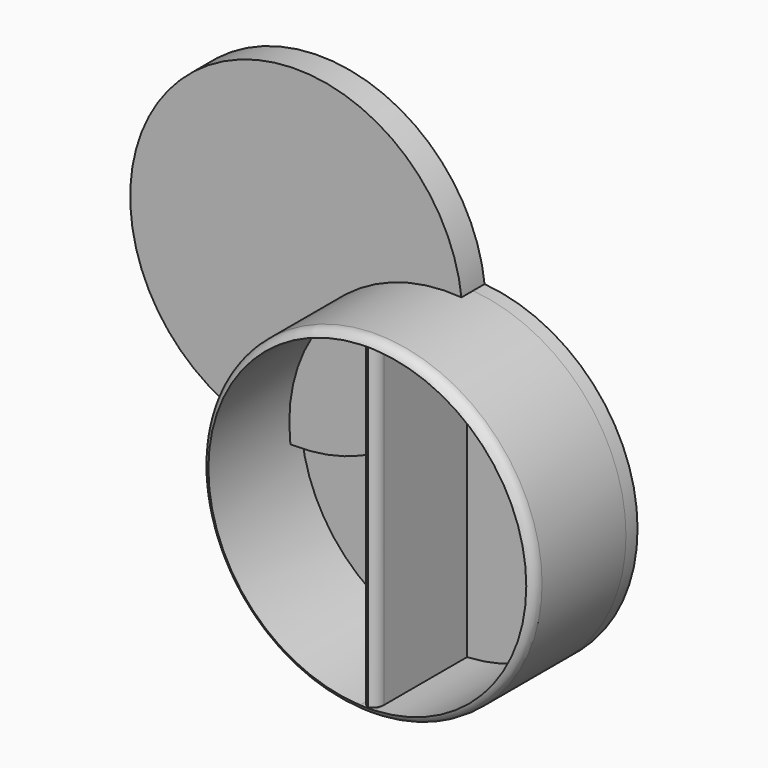
from build123d import *

# Parameters (mm, degrees)
F0_R          = 73.025
F1_DEPTH      = 57.15
F0_W          = 6.35
F0_H          = 139.5556071966
F2_R          = 73.025
F3_DEPTH      = 6.35
F4_2_T1_DEPTH = 164.9556071966
F5_R          = 73.025
F6_DEPTH      = 12.7


# Not quite as in the source:
# - a fillet or chamfer that OpenCascade refuses, or shapes differently, is made with other operations: its cross-section is extruded or revolved along the edge and cut away or added


with BuildPart() as f1:
    # F0 (on Front) → F1 (new body)
    with BuildSketch(Plane.XZ):
        Circle(F0_R)
        with BuildLine():
            ThreePointArc((3.175, 69.7778035983), (50.5014665629, 48.2558221876), (69.85, 0))
            ThreePointArc((69.85, 0), (50.5014665629, -48.2558221876), (3.175, -69.7778035983))
            ThreePointArc((3.175, -69.7778035983), (0, -69.85), (-3.175, -69.7778035983))
            ThreePointArc((-3.175, -69.7778035983), (-69.85, 0), (-3.175, 69.7778035983))
            ThreePointArc((-3.175, 69.7778035983), (0, 69.85), (3.175, 69.7778035983))
        make_face(mode=Mode.SUBTRACT)
    extrude(amount=F1_DEPTH)

    # F4: fillet of radius 5.08 on 1 edges, made by hand

    # F4_s1 → F4_t2 (revolve, cut)
    with BuildSketch(Plane.XY):
        with BuildLine():
            ThreePointArc((73.025, -52.4407139607), (72.1571134838, -55.2805202921), (69.85, -57.15))
            Line((69.85, -57.15), (73.025, -57.15))
            Line((73.025, -57.15), (73.025, -52.4407139607))
        make_face()
    revolve(axis=Axis((0, -57.15, 0), (0, -1, 0)), mode=Mode.SUBTRACT)


with BuildPart() as f1b:
    # F0 (on Front) → F1, piece 2 (new body)
    with BuildSketch(Plane.XZ):
        Rectangle(F0_W, F0_H)
    extrude(amount=F1_DEPTH)

    # F4#2: fillet of radius 5.08 on 2 edges, made by hand

    # F4_2_s2 → F4_2_t1 (cut)
    with BuildSketch(Plane.XY.offset(-82.4778035983)):
        with BuildLine():
            ThreePointArc((-3.175, -52.07), (-1.6871024484, -55.6621024484), (1.905, -57.15))
            Line((1.905, -57.15), (-3.175, -57.15))
            Line((-3.175, -57.15), (-3.175, -52.07))
        make_face()
        with BuildLine():
            ThreePointArc((3.175, -52.07), (1.6871024484, -55.6621024484), (-1.905, -57.15))
            Line((-1.905, -57.15), (3.175, -57.15))
            Line((3.175, -57.15), (3.175, -52.07))
        make_face()
    extrude(amount=F4_2_T1_DEPTH, mode=Mode.SUBTRACT)


with BuildPart() as f3:
    # F2 (on Front) → F3 (new body)
    with BuildSketch(Plane.XZ):
        Circle(F2_R)
    extrude(amount=F3_DEPTH)


with BuildPart() as f6:
    # F5 (on Front) → F6 (new body)
    with BuildSketch(Plane.XZ):
        with Locations((-66.7364522815, 64.5241960883)):
            Circle(F5_R)
    extrude(amount=F6_DEPTH)


solid = Compound([f1.part, f1b.part, f3.part, f6.part])
